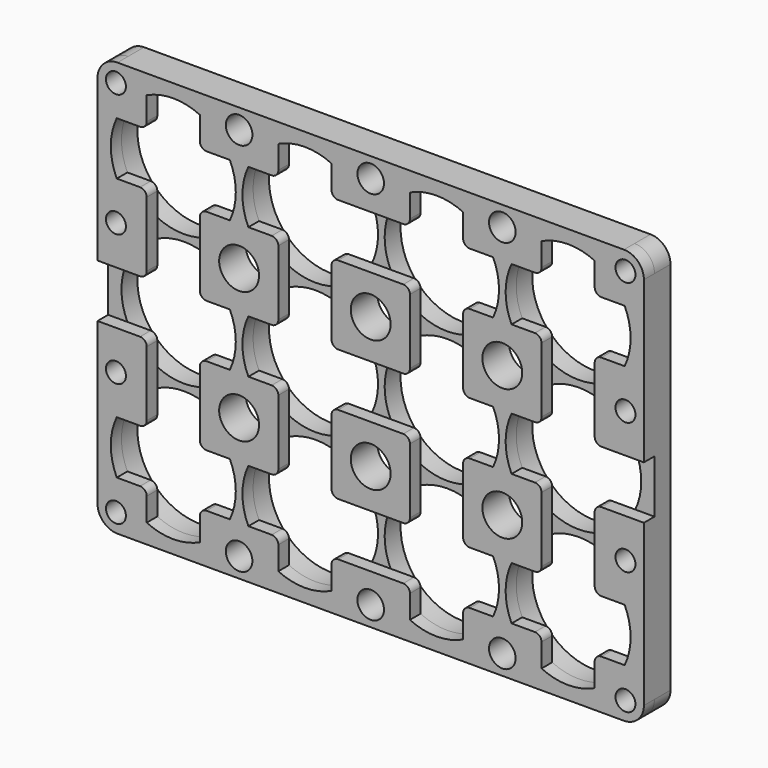
from build123d import *

# Parameters (mm, degrees)
F0_W     = 82.2
F0_H     = 62.4
F0_R     = 1.5
F0_R_2   = 9.4
F0_R_3   = 2
F0_R_4   = 3
F1_DEPTH = 3
F2_R     = 3
F3_R     = 1.5
F3_R_2   = 2
F3_R_3   = 3
F4_DEPTH = 2
F5_R     = 1


# Not quite as in the source:
# - after a boolean that leaves OpenCascade's solid faulty, fix() repairs it


with BuildPart() as f1:
    # F0 (on Front) → F1 (new body)
    with BuildSketch(Plane.XZ):
        with Locations((29.7, 19.8)):
            Rectangle(F0_W, F0_H)
        with Locations((-8.630645927, -8.630645927)):
            Circle(F0_R, mode=Mode.SUBTRACT)
        Circle(F0_R_2, mode=Mode.SUBTRACT)
        with Locations((9.9, -8.4255563615)):
            Circle(F0_R_3, mode=Mode.SUBTRACT)
        with Locations((19.8, 0)):
            Circle(F0_R_2, mode=Mode.SUBTRACT)
        with Locations((-8.630645927, 9.9)):
            Circle(F0_R, mode=Mode.SUBTRACT)
        with Locations((9.9, 9.9)):
            Circle(F0_R_4, mode=Mode.SUBTRACT)
        with Locations((29.7, -8.4255563615)):
            Circle(F0_R_3, mode=Mode.SUBTRACT)
        with Locations((49.5, -8.4255563615)):
            Circle(F0_R_3, mode=Mode.SUBTRACT)
        with Locations((39.6, 0)):
            Circle(F0_R_2, mode=Mode.SUBTRACT)
        with Locations((68.030645927, -8.630645927)):
            Circle(F0_R, mode=Mode.SUBTRACT)
        with Locations((59.4, 0)):
            Circle(F0_R_2, mode=Mode.SUBTRACT)
        with Locations((29.7, 9.9)):
            Circle(F0_R_4, mode=Mode.SUBTRACT)
        with Locations((49.5, 9.9)):
            Circle(F0_R_4, mode=Mode.SUBTRACT)
        with Locations((68.030645927, 9.9)):
            Circle(F0_R, mode=Mode.SUBTRACT)
        with Locations((0, 19.8)):
            Circle(F0_R_2, mode=Mode.SUBTRACT)
        with Locations((-8.630645927, 29.7)):
            Circle(F0_R, mode=Mode.SUBTRACT)
        with Locations((19.8, 19.8)):
            Circle(F0_R_2, mode=Mode.SUBTRACT)
        with Locations((9.9, 29.7)):
            Circle(F0_R_4, mode=Mode.SUBTRACT)
        with Locations((0, 39.6)):
            Circle(F0_R_2, mode=Mode.SUBTRACT)
        with Locations((-8.630645927, 48.230645927)):
            Circle(F0_R, mode=Mode.SUBTRACT)
        with Locations((19.8, 39.6)):
            Circle(F0_R_2, mode=Mode.SUBTRACT)
        with Locations((9.9, 48.0255563615)):
            Circle(F0_R_3, mode=Mode.SUBTRACT)
        with Locations((39.6, 19.8)):
            Circle(F0_R_2, mode=Mode.SUBTRACT)
        with Locations((29.7, 29.7)):
            Circle(F0_R_4, mode=Mode.SUBTRACT)
        with Locations((49.5, 29.7)):
            Circle(F0_R_4, mode=Mode.SUBTRACT)
        with Locations((59.4, 19.8)):
            Circle(F0_R_2, mode=Mode.SUBTRACT)
        with Locations((68.030645927, 29.7)):
            Circle(F0_R, mode=Mode.SUBTRACT)
        with Locations((39.6, 39.6)):
            Circle(F0_R_2, mode=Mode.SUBTRACT)
        with Locations((29.7, 48.0255563615)):
            Circle(F0_R_3, mode=Mode.SUBTRACT)
        with Locations((49.5, 48.0255563615)):
            Circle(F0_R_3, mode=Mode.SUBTRACT)
        with Locations((59.4, 39.6)):
            Circle(F0_R_2, mode=Mode.SUBTRACT)
        with Locations((68.030645927, 48.230645927)):
            Circle(F0_R, mode=Mode.SUBTRACT)
    extrude(amount=F1_DEPTH)

    # F2
    f2_edges = [f1.edges().sort_by_distance(p)[0] for p in [
        (70.8, -1.5, 51),
        (-11.4, -1.5, 51),
        (-11.4, -1.5, -11.4),
        (70.8, -1.5, -11.4),
    ]]
    fillet(f2_edges, radius=F2_R)

    # F3 (on face) → F4 (join)
    with BuildSketch(Plane.XZ.offset(3)):
        with BuildLine():
            ThreePointArc((70.8, 48), (69.9213203436, 50.1213203436), (67.8, 51))
            Line((67.8, 51), (63.4, 51))
            Line((63.4, 51), (63.4, 48.1064681273))
            ThreePointArc((63.4, 48.1064681273), (66.0468037432, 46.2468037432), (67.9064681273, 43.6))
            Line((67.9064681273, 43.6), (70.8, 43.6))
            Line((70.8, 43.6), (70.8, 48))
        make_face()
        with Locations((68.030645927, 48.230645927)):
            Circle(F3_R, mode=Mode.SUBTRACT)
        with BuildLine():
            Line((63.4, 48.1064681273), (63.4, 51))
            Line((63.4, 51), (55.4, 51))
            Line((55.4, 51), (55.4, 48.1064681273))
            ThreePointArc((55.4, 48.1064681273), (59.4, 49), (63.4, 48.1064681273))
        make_face()
        with BuildLine():
            Line((55.4, 48.1064681273), (55.4, 51))
            Line((55.4, 51), (43.6, 51))
            Line((43.6, 51), (43.6, 48.1064681273))
            ThreePointArc((43.6, 48.1064681273), (46.2468037432, 46.2468037432), (48.1064681273, 43.6))
            Line((48.1064681273, 43.6), (50.8935318727, 43.6))
            ThreePointArc((50.8935318727, 43.6), (52.7531962568, 46.2468037432), (55.4, 48.1064681273))
        make_face()
        with Locations((49.5, 48.0255563615)):
            Circle(F3_R_2, mode=Mode.SUBTRACT)
        with BuildLine():
            ThreePointArc((67.9064681273, 43.6), (66.0468037432, 46.2468037432), (63.4, 48.1064681273))
            Line((63.4, 48.1064681273), (63.4, 43.6))
            Line((63.4, 43.6), (67.9064681273, 43.6))
        make_face()
        with BuildLine():
            Line((70.8, 39.6), (70.8, 43.6))
            Line((70.8, 43.6), (67.9064681273, 43.6))
            ThreePointArc((67.9064681273, 43.6), (68.5738977648, 41.6492925125), (68.8, 39.6))
            ThreePointArc((68.8, 39.6), (68.5738977648, 37.5507074875), (67.9064681273, 35.6))
            Line((67.9064681273, 35.6), (70.8, 35.6))
            Line((70.8, 35.6), (70.8, 39.6))
        make_face()
        with BuildLine():
            Line((43.6, 48.1064681273), (43.6, 51))
            Line((43.6, 51), (35.6, 51))
            Line((35.6, 51), (35.6, 48.1064681273))
            ThreePointArc((35.6, 48.1064681273), (39.6, 49), (43.6, 48.1064681273))
        make_face()
        with BuildLine():
            Line((55.4, 43.6), (55.4, 48.1064681273))
            ThreePointArc((55.4, 48.1064681273), (52.7531962568, 46.2468037432), (50.8935318727, 43.6))
            Line((50.8935318727, 43.6), (55.4, 43.6))
        make_face()
        with BuildLine():
            Line((35.6, 48.1064681273), (35.6, 51))
            Line((35.6, 51), (23.8, 51))
            Line((23.8, 51), (23.8, 48.1064681273))
            ThreePointArc((23.8, 48.1064681273), (26.4468037432, 46.2468037432), (28.3064681273, 43.6))
            Line((28.3064681273, 43.6), (31.0935318727, 43.6))
            ThreePointArc((31.0935318727, 43.6), (32.9531962568, 46.2468037432), (35.6, 48.1064681273))
        make_face()
        with Locations((29.7, 48.0255563615)):
            Circle(F3_R_2, mode=Mode.SUBTRACT)
        with BuildLine():
            ThreePointArc((48.1064681273, 43.6), (46.2468037432, 46.2468037432), (43.6, 48.1064681273))
            Line((43.6, 48.1064681273), (43.6, 43.6))
            Line((43.6, 43.6), (48.1064681273, 43.6))
        make_face()
        with BuildLine():
            ThreePointArc((50.8935318727, 35.6), (50, 39.6), (50.8935318727, 43.6))
            Line((50.8935318727, 43.6), (48.1064681273, 43.6))
            ThreePointArc((48.1064681273, 43.6), (48.7738977648, 41.6492925125), (49, 39.6))
            ThreePointArc((49, 39.6), (48.7738977648, 37.5507074875), (48.1064681273, 35.6))
            Line((48.1064681273, 35.6), (50.8935318727, 35.6))
        make_face()
        with BuildLine():
            Line((70.8, 23.8), (70.8, 35.6))
            Line((70.8, 35.6), (67.9064681273, 35.6))
            ThreePointArc((67.9064681273, 35.6), (66.0468037432, 32.9531962568), (63.4, 31.0935318727))
            Line((63.4, 31.0935318727), (63.4, 28.3064681273))
            ThreePointArc((63.4, 28.3064681273), (66.0468037432, 26.4468037432), (67.9064681273, 23.8))
            Line((67.9064681273, 23.8), (70.8, 23.8))
        make_face()
        with Locations((68.030645927, 29.7)):
            Circle(F3_R, mode=Mode.SUBTRACT)
        with BuildLine():
            Line((23.8, 48.1064681273), (23.8, 51))
            Line((23.8, 51), (15.8, 51))
            Line((15.8, 51), (15.8, 48.1064681273))
            ThreePointArc((15.8, 48.1064681273), (19.8, 49), (23.8, 48.1064681273))
        make_face()
        with BuildLine():
            Line((35.6, 43.6), (35.6, 48.1064681273))
            ThreePointArc((35.6, 48.1064681273), (32.9531962568, 46.2468037432), (31.0935318727, 43.6))
            Line((31.0935318727, 43.6), (35.6, 43.6))
        make_face()
        with BuildLine():
            Line((55.4, 35.6), (50.8935318727, 35.6))
            ThreePointArc((50.8935318727, 35.6), (52.7531962568, 32.9531962568), (55.4, 31.0935318727))
            Line((55.4, 31.0935318727), (55.4, 35.6))
        make_face()
        with BuildLine():
            ThreePointArc((55.4, 31.0935318727), (52.7531962568, 32.9531962568), (50.8935318727, 35.6))
            Line((50.8935318727, 35.6), (48.1064681273, 35.6))
            ThreePointArc((48.1064681273, 35.6), (46.2468037432, 32.9531962568), (43.6, 31.0935318727))
            Line((43.6, 31.0935318727), (43.6, 28.3064681273))
            ThreePointArc((43.6, 28.3064681273), (46.2468037432, 26.4468037432), (48.1064681273, 23.8))
            Line((48.1064681273, 23.8), (50.8935318727, 23.8))
            ThreePointArc((50.8935318727, 23.8), (52.7531962568, 26.4468037432), (55.4, 28.3064681273))
            Line((55.4, 28.3064681273), (55.4, 31.0935318727))
        make_face()
        with Locations((49.5, 29.7)):
            Circle(F3_R_3, mode=Mode.SUBTRACT)
        with BuildLine():
            ThreePointArc((63.4, 31.0935318727), (66.0468037432, 32.9531962568), (67.9064681273, 35.6))
            Line((67.9064681273, 35.6), (63.4, 35.6))
            Line((63.4, 35.6), (63.4, 31.0935318727))
        make_face()
        with BuildLine():
            Line((15.8, 48.1064681273), (15.8, 51))
            Line((15.8, 51), (4, 51))
            Line((4, 51), (4, 48.1064681273))
            ThreePointArc((4, 48.1064681273), (6.6468037432, 46.2468037432), (8.5064681273, 43.6))
            Line((8.5064681273, 43.6), (11.2935318727, 43.6))
            ThreePointArc((11.2935318727, 43.6), (13.1531962568, 46.2468037432), (15.8, 48.1064681273))
        make_face()
        with Locations((9.9, 48.0255563615)):
            Circle(F3_R_2, mode=Mode.SUBTRACT)
        with BuildLine():
            ThreePointArc((28.3064681273, 43.6), (26.4468037432, 46.2468037432), (23.8, 48.1064681273))
            Line((23.8, 48.1064681273), (23.8, 43.6))
            Line((23.8, 43.6), (28.3064681273, 43.6))
        make_face()
        with BuildLine():
            ThreePointArc((43.6, 31.0935318727), (46.2468037432, 32.9531962568), (48.1064681273, 35.6))
            Line((48.1064681273, 35.6), (43.6, 35.6))
            Line((43.6, 35.6), (43.6, 31.0935318727))
        make_face()
        with BuildLine():
            Line((70.8, 4), (70.8, 15.8))
            Line((70.8, 15.8), (67.9064681273, 15.8))
            ThreePointArc((67.9064681273, 15.8), (66.0468037432, 13.1531962568), (63.4, 11.2935318727))
            Line((63.4, 11.2935318727), (63.4, 8.5064681273))
            ThreePointArc((63.4, 8.5064681273), (66.0468037432, 6.6468037432), (67.9064681273, 4))
            Line((67.9064681273, 4), (70.8, 4))
        make_face()
        with Locations((68.030645927, 9.9)):
            Circle(F3_R, mode=Mode.SUBTRACT)
        with BuildLine():
            Line((63.4, 23.8), (67.9064681273, 23.8))
            ThreePointArc((67.9064681273, 23.8), (66.0468037432, 26.4468037432), (63.4, 28.3064681273))
            Line((63.4, 28.3064681273), (63.4, 23.8))
        make_face()
        with BuildLine():
            Line((4, 48.1064681273), (4, 51))
            Line((4, 51), (-4, 51))
            Line((-4, 51), (-4, 48.1064681273))
            ThreePointArc((-4, 48.1064681273), (0, 49), (4, 48.1064681273))
        make_face()
        with BuildLine():
            Line((15.8, 43.6), (15.8, 48.1064681273))
            ThreePointArc((15.8, 48.1064681273), (13.1531962568, 46.2468037432), (11.2935318727, 43.6))
            Line((11.2935318727, 43.6), (15.8, 43.6))
        make_face()
        with BuildLine():
            Line((35.6, 35.6), (31.0935318727, 35.6))
            ThreePointArc((31.0935318727, 35.6), (32.9531962568, 32.9531962568), (35.6, 31.0935318727))
            Line((35.6, 31.0935318727), (35.6, 35.6))
        make_face()
        with BuildLine():
            ThreePointArc((35.6, 31.0935318727), (32.9531962568, 32.9531962568), (31.0935318727, 35.6))
            Line((31.0935318727, 35.6), (28.3064681273, 35.6))
            ThreePointArc((28.3064681273, 35.6), (26.4468037432, 32.9531962568), (23.8, 31.0935318727))
            Line((23.8, 31.0935318727), (23.8, 28.3064681273))
            ThreePointArc((23.8, 28.3064681273), (26.4468037432, 26.4468037432), (28.3064681273, 23.8))
            Line((28.3064681273, 23.8), (31.0935318727, 23.8))
            ThreePointArc((31.0935318727, 23.8), (32.9531962568, 26.4468037432), (35.6, 28.3064681273))
            Line((35.6, 28.3064681273), (35.6, 31.0935318727))
        make_face()
        with Locations((29.7, 29.7)):
            Circle(F3_R_3, mode=Mode.SUBTRACT)
        with BuildLine():
            Line((55.4, 23.8), (55.4, 28.3064681273))
            ThreePointArc((55.4, 28.3064681273), (52.7531962568, 26.4468037432), (50.8935318727, 23.8))
            Line((50.8935318727, 23.8), (55.4, 23.8))
        make_face()
        with BuildLine():
            Line((70.8, -4), (70.8, 4))
            Line((70.8, 4), (67.9064681273, 4))
            ThreePointArc((67.9064681273, 4), (68.5738977648, 2.0492925125), (68.8, 0))
            ThreePointArc((68.8, 0), (68.5738977648, -2.0492925125), (67.9064681273, -4))
            Line((67.9064681273, -4), (70.8, -4))
        make_face()
        with BuildLine():
            ThreePointArc((63.4, 11.2935318727), (66.0468037432, 13.1531962568), (67.9064681273, 15.8))
            Line((67.9064681273, 15.8), (63.4, 15.8))
            Line((63.4, 15.8), (63.4, 11.2935318727))
        make_face()
        with BuildLine():
            Line((-4, 48.1064681273), (-4, 51))
            Line((-4, 51), (-8.4, 51))
            ThreePointArc((-8.4, 51), (-10.5213203436, 50.1213203436), (-11.4, 48))
            Line((-11.4, 48), (-11.4, 43.6))
            Line((-11.4, 43.6), (-8.5064681273, 43.6))
            ThreePointArc((-8.5064681273, 43.6), (-6.6468037432, 46.2468037432), (-4, 48.1064681273))
        make_face()
        with Locations((-8.630645927, 48.230645927)):
            Circle(F3_R, mode=Mode.SUBTRACT)
        with BuildLine():
            ThreePointArc((8.5064681273, 43.6), (6.6468037432, 46.2468037432), (4, 48.1064681273))
            Line((4, 48.1064681273), (4, 43.6))
            Line((4, 43.6), (8.5064681273, 43.6))
        make_face()
        with BuildLine():
            ThreePointArc((11.2935318727, 35.6), (10.4, 39.6), (11.2935318727, 43.6))
            Line((11.2935318727, 43.6), (8.5064681273, 43.6))
            ThreePointArc((8.5064681273, 43.6), (9.1738977648, 41.6492925125), (9.4, 39.6))
            ThreePointArc((9.4, 39.6), (9.1738977648, 37.5507074875), (8.5064681273, 35.6))
            Line((8.5064681273, 35.6), (11.2935318727, 35.6))
        make_face()
        with BuildLine():
            ThreePointArc((23.8, 31.0935318727), (26.4468037432, 32.9531962568), (28.3064681273, 35.6))
            Line((28.3064681273, 35.6), (23.8, 35.6))
            Line((23.8, 35.6), (23.8, 31.0935318727))
        make_face()
        with BuildLine():
            ThreePointArc((50.8935318727, 15.8), (50, 19.8), (50.8935318727, 23.8))
            Line((50.8935318727, 23.8), (48.1064681273, 23.8))
            ThreePointArc((48.1064681273, 23.8), (48.7738977648, 21.8492925125), (49, 19.8))
            ThreePointArc((49, 19.8), (48.7738977648, 17.7507074875), (48.1064681273, 15.8))
            Line((48.1064681273, 15.8), (50.8935318727, 15.8))
        make_face()
        with BuildLine():
            ThreePointArc((48.1064681273, 23.8), (46.2468037432, 26.4468037432), (43.6, 28.3064681273))
            Line((43.6, 28.3064681273), (43.6, 23.8))
            Line((43.6, 23.8), (48.1064681273, 23.8))
        make_face()
        with BuildLine():
            Line((70.8, -8.4), (70.8, -4))
            Line((70.8, -4), (67.9064681273, -4))
            ThreePointArc((67.9064681273, -4), (66.0468037432, -6.6468037432), (63.4, -8.5064681273))
            Line((63.4, -8.5064681273), (63.4, -11.4))
            Line((63.4, -11.4), (67.8, -11.4))
            ThreePointArc((67.8, -11.4), (69.9213203436, -10.5213203436), (70.8, -8.4))
        make_face()
        with Locations((68.030645927, -8.630645927)):
            Circle(F3_R, mode=Mode.SUBTRACT)
        with BuildLine():
            Line((63.4, 4), (67.9064681273, 4))
            ThreePointArc((67.9064681273, 4), (66.0468037432, 6.6468037432), (63.4, 8.5064681273))
            Line((63.4, 8.5064681273), (63.4, 4))
        make_face()
        with BuildLine():
            Line((-4, 43.6), (-4, 48.1064681273))
            ThreePointArc((-4, 48.1064681273), (-6.6468037432, 46.2468037432), (-8.5064681273, 43.6))
            Line((-8.5064681273, 43.6), (-4, 43.6))
        make_face()
        with BuildLine():
            Line((15.8, 35.6), (11.2935318727, 35.6))
            ThreePointArc((11.2935318727, 35.6), (13.1531962568, 32.9531962568), (15.8, 31.0935318727))
            Line((15.8, 31.0935318727), (15.8, 35.6))
        make_face()
        with BuildLine():
            ThreePointArc((15.8, 31.0935318727), (13.1531962568, 32.9531962568), (11.2935318727, 35.6))
            Line((11.2935318727, 35.6), (8.5064681273, 35.6))
            ThreePointArc((8.5064681273, 35.6), (6.6468037432, 32.9531962568), (4, 31.0935318727))
            Line((4, 31.0935318727), (4, 28.3064681273))
            ThreePointArc((4, 28.3064681273), (6.6468037432, 26.4468037432), (8.5064681273, 23.8))
            Line((8.5064681273, 23.8), (11.2935318727, 23.8))
            ThreePointArc((11.2935318727, 23.8), (13.1531962568, 26.4468037432), (15.8, 28.3064681273))
            Line((15.8, 28.3064681273), (15.8, 31.0935318727))
        make_face()
        with Locations((9.9, 29.7)):
            Circle(F3_R_3, mode=Mode.SUBTRACT)
        with BuildLine():
            Line((35.6, 23.8), (35.6, 28.3064681273))
            ThreePointArc((35.6, 28.3064681273), (32.9531962568, 26.4468037432), (31.0935318727, 23.8))
            Line((31.0935318727, 23.8), (35.6, 23.8))
        make_face()
        with BuildLine():
            Line((55.4, 15.8), (50.8935318727, 15.8))
            ThreePointArc((50.8935318727, 15.8), (52.7531962568, 13.1531962568), (55.4, 11.2935318727))
            Line((55.4, 11.2935318727), (55.4, 15.8))
        make_face()
        with BuildLine():
            ThreePointArc((55.4, 11.2935318727), (52.7531962568, 13.1531962568), (50.8935318727, 15.8))
            Line((50.8935318727, 15.8), (48.1064681273, 15.8))
            ThreePointArc((48.1064681273, 15.8), (46.2468037432, 13.1531962568), (43.6, 11.2935318727))
            Line((43.6, 11.2935318727), (43.6, 8.5064681273))
            ThreePointArc((43.6, 8.5064681273), (46.2468037432, 6.6468037432), (48.1064681273, 4))
            Line((48.1064681273, 4), (50.8935318727, 4))
            ThreePointArc((50.8935318727, 4), (52.7531962568, 6.6468037432), (55.4, 8.5064681273))
            Line((55.4, 8.5064681273), (55.4, 11.2935318727))
        make_face()
        with Locations((49.5, 9.9)):
            Circle(F3_R_3, mode=Mode.SUBTRACT)
        with BuildLine():
            ThreePointArc((63.4, -8.5064681273), (66.0468037432, -6.6468037432), (67.9064681273, -4))
            Line((67.9064681273, -4), (63.4, -4))
            Line((63.4, -4), (63.4, -8.5064681273))
        make_face()
        with BuildLine():
            ThreePointArc((-8.5064681273, 35.6), (-9.4, 39.6), (-8.5064681273, 43.6))
            Line((-8.5064681273, 43.6), (-11.4, 43.6))
            Line((-11.4, 43.6), (-11.4, 39.6))
            Line((-11.4, 39.6), (-11.4, 35.6))
            Line((-11.4, 35.6), (-8.5064681273, 35.6))
        make_face()
        with BuildLine():
            ThreePointArc((4, 31.0935318727), (6.6468037432, 32.9531962568), (8.5064681273, 35.6))
            Line((8.5064681273, 35.6), (4, 35.6))
            Line((4, 35.6), (4, 31.0935318727))
        make_face()
        with BuildLine():
            ThreePointArc((28.3064681273, 23.8), (26.4468037432, 26.4468037432), (23.8, 28.3064681273))
            Line((23.8, 28.3064681273), (23.8, 23.8))
            Line((23.8, 23.8), (28.3064681273, 23.8))
        make_face()
        with BuildLine():
            ThreePointArc((43.6, 11.2935318727), (46.2468037432, 13.1531962568), (48.1064681273, 15.8))
            Line((48.1064681273, 15.8), (43.6, 15.8))
            Line((43.6, 15.8), (43.6, 11.2935318727))
        make_face()
        with BuildLine():
            Line((63.4, -11.4), (63.4, -8.5064681273))
            ThreePointArc((63.4, -8.5064681273), (59.4, -9.4), (55.4, -8.5064681273))
            Line((55.4, -8.5064681273), (55.4, -11.4))
            Line((55.4, -11.4), (63.4, -11.4))
        make_face()
        with BuildLine():
            Line((55.4, 4), (55.4, 8.5064681273))
            ThreePointArc((55.4, 8.5064681273), (52.7531962568, 6.6468037432), (50.8935318727, 4))
            Line((50.8935318727, 4), (55.4, 4))
        make_face()
        with BuildLine():
            ThreePointArc((-4, 31.0935318727), (-6.6468037432, 32.9531962568), (-8.5064681273, 35.6))
            Line((-8.5064681273, 35.6), (-11.4, 35.6))
            Line((-11.4, 35.6), (-11.4, 23.8))
            Line((-11.4, 23.8), (-8.5064681273, 23.8))
            ThreePointArc((-8.5064681273, 23.8), (-6.6468037432, 26.4468037432), (-4, 28.3064681273))
            Line((-4, 28.3064681273), (-4, 31.0935318727))
        make_face()
        with Locations((-8.630645927, 29.7)):
            Circle(F3_R, mode=Mode.SUBTRACT)
        with BuildLine():
            Line((-4, 35.6), (-8.5064681273, 35.6))
            ThreePointArc((-8.5064681273, 35.6), (-6.6468037432, 32.9531962568), (-4, 31.0935318727))
            Line((-4, 31.0935318727), (-4, 35.6))
        make_face()
        with BuildLine():
            Line((15.8, 23.8), (15.8, 28.3064681273))
            ThreePointArc((15.8, 28.3064681273), (13.1531962568, 26.4468037432), (11.2935318727, 23.8))
            Line((11.2935318727, 23.8), (15.8, 23.8))
        make_face()
        with BuildLine():
            Line((35.6, 15.8), (31.0935318727, 15.8))
            ThreePointArc((31.0935318727, 15.8), (32.9531962568, 13.1531962568), (35.6, 11.2935318727))
            Line((35.6, 11.2935318727), (35.6, 15.8))
        make_face()
        with BuildLine():
            ThreePointArc((35.6, 11.2935318727), (32.9531962568, 13.1531962568), (31.0935318727, 15.8))
            Line((31.0935318727, 15.8), (28.3064681273, 15.8))
            ThreePointArc((28.3064681273, 15.8), (26.4468037432, 13.1531962568), (23.8, 11.2935318727))
            Line((23.8, 11.2935318727), (23.8, 8.5064681273))
            ThreePointArc((23.8, 8.5064681273), (26.4468037432, 6.6468037432), (28.3064681273, 4))
            Line((28.3064681273, 4), (31.0935318727, 4))
            ThreePointArc((31.0935318727, 4), (32.9531962568, 6.6468037432), (35.6, 8.5064681273))
            Line((35.6, 8.5064681273), (35.6, 11.2935318727))
        make_face()
        with Locations((29.7, 9.9)):
            Circle(F3_R_3, mode=Mode.SUBTRACT)
        with BuildLine():
            Line((55.4, -11.4), (55.4, -8.5064681273))
            ThreePointArc((55.4, -8.5064681273), (52.7531962568, -6.6468037432), (50.8935318727, -4))
            Line((50.8935318727, -4), (48.1064681273, -4))
            ThreePointArc((48.1064681273, -4), (46.2468037432, -6.6468037432), (43.6, -8.5064681273))
            Line((43.6, -8.5064681273), (43.6, -11.4))
            Line((43.6, -11.4), (55.4, -11.4))
        make_face()
        with Locations((49.5, -8.4255563615)):
            Circle(F3_R_2, mode=Mode.SUBTRACT)
        with BuildLine():
            ThreePointArc((50.8935318727, -4), (52.7531962568, -6.6468037432), (55.4, -8.5064681273))
            Line((55.4, -8.5064681273), (55.4, -4))
            Line((55.4, -4), (50.8935318727, -4))
        make_face()
        with BuildLine():
            ThreePointArc((50.8935318727, -4), (50, 0), (50.8935318727, 4))
            Line((50.8935318727, 4), (48.1064681273, 4))
            ThreePointArc((48.1064681273, 4), (48.7738977648, 2.0492925125), (49, 0))
            ThreePointArc((49, 0), (48.7738977648, -2.0492925125), (48.1064681273, -4))
            Line((48.1064681273, -4), (50.8935318727, -4))
        make_face()
        with BuildLine():
            ThreePointArc((11.2935318727, 15.8), (10.4, 19.8), (11.2935318727, 23.8))
            Line((11.2935318727, 23.8), (8.5064681273, 23.8))
            ThreePointArc((8.5064681273, 23.8), (9.1738977648, 21.8492925125), (9.4, 19.8))
            ThreePointArc((9.4, 19.8), (9.1738977648, 17.7507074875), (8.5064681273, 15.8))
            Line((8.5064681273, 15.8), (11.2935318727, 15.8))
        make_face()
        with BuildLine():
            ThreePointArc((8.5064681273, 23.8), (6.6468037432, 26.4468037432), (4, 28.3064681273))
            Line((4, 28.3064681273), (4, 23.8))
            Line((4, 23.8), (8.5064681273, 23.8))
        make_face()
        with BuildLine():
            ThreePointArc((23.8, 11.2935318727), (26.4468037432, 13.1531962568), (28.3064681273, 15.8))
            Line((28.3064681273, 15.8), (23.8, 15.8))
            Line((23.8, 15.8), (23.8, 11.2935318727))
        make_face()
        with BuildLine():
            ThreePointArc((48.1064681273, 4), (46.2468037432, 6.6468037432), (43.6, 8.5064681273))
            Line((43.6, 8.5064681273), (43.6, 4))
            Line((43.6, 4), (48.1064681273, 4))
        make_face()
        with BuildLine():
            Line((-4, 23.8), (-4, 28.3064681273))
            ThreePointArc((-4, 28.3064681273), (-6.6468037432, 26.4468037432), (-8.5064681273, 23.8))
            Line((-8.5064681273, 23.8), (-4, 23.8))
        make_face()
        with BuildLine():
            Line((15.8, 15.8), (11.2935318727, 15.8))
            ThreePointArc((11.2935318727, 15.8), (13.1531962568, 13.1531962568), (15.8, 11.2935318727))
            Line((15.8, 11.2935318727), (15.8, 15.8))
        make_face()
        with BuildLine():
            ThreePointArc((15.8, 11.2935318727), (13.1531962568, 13.1531962568), (11.2935318727, 15.8))
            Line((11.2935318727, 15.8), (8.5064681273, 15.8))
            ThreePointArc((8.5064681273, 15.8), (6.6468037432, 13.1531962568), (4, 11.2935318727))
            Line((4, 11.2935318727), (4, 8.5064681273))
            ThreePointArc((4, 8.5064681273), (6.6468037432, 6.6468037432), (8.5064681273, 4))
            Line((8.5064681273, 4), (11.2935318727, 4))
            ThreePointArc((11.2935318727, 4), (13.1531962568, 6.6468037432), (15.8, 8.5064681273))
            Line((15.8, 8.5064681273), (15.8, 11.2935318727))
        make_face()
        with Locations((9.9, 9.9)):
            Circle(F3_R_3, mode=Mode.SUBTRACT)
        with BuildLine():
            Line((35.6, 4), (35.6, 8.5064681273))
            ThreePointArc((35.6, 8.5064681273), (32.9531962568, 6.6468037432), (31.0935318727, 4))
            Line((31.0935318727, 4), (35.6, 4))
        make_face()
        with BuildLine():
            Line((35.6, -11.4), (43.6, -11.4))
            Line((43.6, -11.4), (43.6, -8.5064681273))
            ThreePointArc((43.6, -8.5064681273), (39.6, -9.4), (35.6, -8.5064681273))
            Line((35.6, -8.5064681273), (35.6, -11.4))
        make_face()
        with BuildLine():
            ThreePointArc((43.6, -8.5064681273), (46.2468037432, -6.6468037432), (48.1064681273, -4))
            Line((48.1064681273, -4), (43.6, -4))
            Line((43.6, -4), (43.6, -8.5064681273))
        make_face()
        with BuildLine():
            Line((-8.5064681273, 15.8), (-11.4, 15.8))
            Line((-11.4, 15.8), (-11.4, 4))
            Line((-11.4, 4), (-8.5064681273, 4))
            ThreePointArc((-8.5064681273, 4), (-6.6468037432, 6.6468037432), (-4, 8.5064681273))
            Line((-4, 8.5064681273), (-4, 11.2935318727))
            ThreePointArc((-4, 11.2935318727), (-6.6468037432, 13.1531962568), (-8.5064681273, 15.8))
        make_face()
        with Locations((-8.630645927, 9.9)):
            Circle(F3_R, mode=Mode.SUBTRACT)
        with BuildLine():
            ThreePointArc((4, 11.2935318727), (6.6468037432, 13.1531962568), (8.5064681273, 15.8))
            Line((8.5064681273, 15.8), (4, 15.8))
            Line((4, 15.8), (4, 11.2935318727))
        make_face()
        with BuildLine():
            ThreePointArc((28.3064681273, 4), (26.4468037432, 6.6468037432), (23.8, 8.5064681273))
            Line((23.8, 8.5064681273), (23.8, 4))
            Line((23.8, 4), (28.3064681273, 4))
        make_face()
        with BuildLine():
            Line((23.8, -11.4), (35.6, -11.4))
            Line((35.6, -11.4), (35.6, -8.5064681273))
            ThreePointArc((35.6, -8.5064681273), (32.9531962568, -6.6468037432), (31.0935318727, -4))
            Line((31.0935318727, -4), (28.3064681273, -4))
            ThreePointArc((28.3064681273, -4), (26.4468037432, -6.6468037432), (23.8, -8.5064681273))
            Line((23.8, -8.5064681273), (23.8, -11.4))
        make_face()
        with Locations((29.7, -8.4255563615)):
            Circle(F3_R_2, mode=Mode.SUBTRACT)
        with BuildLine():
            Line((-8.5064681273, 4), (-11.4, 4))
            Line((-11.4, 4), (-11.4, -4))
            Line((-11.4, -4), (-8.5064681273, -4))
            ThreePointArc((-8.5064681273, -4), (-9.4, 0), (-8.5064681273, 4))
        make_face()
        with BuildLine():
            Line((-4, 15.8), (-8.5064681273, 15.8))
            ThreePointArc((-8.5064681273, 15.8), (-6.6468037432, 13.1531962568), (-4, 11.2935318727))
            Line((-4, 11.2935318727), (-4, 15.8))
        make_face()
        with BuildLine():
            Line((15.8, 4), (15.8, 8.5064681273))
            ThreePointArc((15.8, 8.5064681273), (13.1531962568, 6.6468037432), (11.2935318727, 4))
            Line((11.2935318727, 4), (15.8, 4))
        make_face()
        with BuildLine():
            Line((35.6, -4), (31.0935318727, -4))
            ThreePointArc((31.0935318727, -4), (32.9531962568, -6.6468037432), (35.6, -8.5064681273))
            Line((35.6, -8.5064681273), (35.6, -4))
        make_face()
        with BuildLine():
            Line((15.8, -11.4), (23.8, -11.4))
            Line((23.8, -11.4), (23.8, -8.5064681273))
            ThreePointArc((23.8, -8.5064681273), (19.8, -9.4), (15.8, -8.5064681273))
            Line((15.8, -8.5064681273), (15.8, -11.4))
        make_face()
        with BuildLine():
            Line((-8.5064681273, -4), (-11.4, -4))
            Line((-11.4, -4), (-11.4, -8.4))
            ThreePointArc((-11.4, -8.4), (-10.5213203436, -10.5213203436), (-8.4, -11.4))
            Line((-8.4, -11.4), (-4, -11.4))
            Line((-4, -11.4), (-4, -8.5064681273))
            ThreePointArc((-4, -8.5064681273), (-6.6468037432, -6.6468037432), (-8.5064681273, -4))
        make_face()
        with Locations((-8.630645927, -8.630645927)):
            Circle(F3_R, mode=Mode.SUBTRACT)
        with BuildLine():
            ThreePointArc((-4, 8.5064681273), (-6.6468037432, 6.6468037432), (-8.5064681273, 4))
            Line((-8.5064681273, 4), (-4, 4))
            Line((-4, 4), (-4, 8.5064681273))
        make_face()
        with BuildLine():
            ThreePointArc((11.2935318727, -4), (10.4, 0), (11.2935318727, 4))
            Line((11.2935318727, 4), (8.5064681273, 4))
            ThreePointArc((8.5064681273, 4), (9.1738977648, 2.0492925125), (9.4, 0))
            ThreePointArc((9.4, 0), (9.1738977648, -2.0492925125), (8.5064681273, -4))
            Line((8.5064681273, -4), (11.2935318727, -4))
        make_face()
        with BuildLine():
            ThreePointArc((8.5064681273, 4), (6.6468037432, 6.6468037432), (4, 8.5064681273))
            Line((4, 8.5064681273), (4, 4))
            Line((4, 4), (8.5064681273, 4))
        make_face()
        with BuildLine():
            ThreePointArc((23.8, -8.5064681273), (26.4468037432, -6.6468037432), (28.3064681273, -4))
            Line((28.3064681273, -4), (23.8, -4))
            Line((23.8, -4), (23.8, -8.5064681273))
        make_face()
        with BuildLine():
            Line((4, -11.4), (15.8, -11.4))
            Line((15.8, -11.4), (15.8, -8.5064681273))
            ThreePointArc((15.8, -8.5064681273), (13.1531962568, -6.6468037432), (11.2935318727, -4))
            Line((11.2935318727, -4), (8.5064681273, -4))
            ThreePointArc((8.5064681273, -4), (6.6468037432, -6.6468037432), (4, -8.5064681273))
            Line((4, -8.5064681273), (4, -11.4))
        make_face()
        with Locations((9.9, -8.4255563615)):
            Circle(F3_R_2, mode=Mode.SUBTRACT)
        with BuildLine():
            Line((-4, -4), (-8.5064681273, -4))
            ThreePointArc((-8.5064681273, -4), (-6.6468037432, -6.6468037432), (-4, -8.5064681273))
            Line((-4, -8.5064681273), (-4, -4))
        make_face()
        with BuildLine():
            Line((15.8, -4), (11.2935318727, -4))
            ThreePointArc((11.2935318727, -4), (13.1531962568, -6.6468037432), (15.8, -8.5064681273))
            Line((15.8, -8.5064681273), (15.8, -4))
        make_face()
        with BuildLine():
            Line((-4, -11.4), (4, -11.4))
            Line((4, -11.4), (4, -8.5064681273))
            ThreePointArc((4, -8.5064681273), (0, -9.4), (-4, -8.5064681273))
            Line((-4, -8.5064681273), (-4, -11.4))
        make_face()
        with BuildLine():
            ThreePointArc((4, -8.5064681273), (6.6468037432, -6.6468037432), (8.5064681273, -4))
            Line((8.5064681273, -4), (4, -4))
            Line((4, -4), (4, -8.5064681273))
        make_face()
    extrude(amount=F4_DEPTH)

    add(f1.part.fix(), mode=Mode.REPLACE)

    # F5
    f5_edges = [f1.edges().sort_by_distance(p)[0] for p in [
        (-4, -4, 43.6),
        (4, -4, 43.6),
        (15.8, -4, 43.6),
        (23.8, -4, 43.6),
        (35.6, -4, 43.6),
        (43.6, -4, 43.6),
        (55.4, -4, 43.6),
        (63.4, -4, 43.6),
        (63.4, -4, 23.8),
        (55.4, -4, 23.8),
        (43.6, -4, 23.8),
        (35.6, -4, 23.8),
        (15.8, -4, 23.8),
        (23.8, -4, 23.8),
        (-4, -4, 23.8),
        (4, -4, 23.8),
        (-4, -4, 15.8),
        (-4, -4, 4),
        (4, -4, 4),
        (15.8, -4, 4),
        (15.8, -4, 15.8),
        (23.8, -4, 4),
        (35.6, -4, 4),
        (35.6, -4, 15.8),
        (43.6, -4, 4),
        (55.4, -4, 4),
        (63.4, -4, 4),
        (55.4, -4, 15.8),
        (55.4, -4, -4),
        (-4, -4, -4),
        (4, -4, -4),
        (15.8, -4, -4),
        (23.8, -4, -4),
        (35.6, -4, -4),
        (43.6, -4, -4),
        (63.4, -4, -4),
        (63.4, -4, 15.8),
        (43.6, -4, 15.8),
        (23.8, -4, 15.8),
        (4, -4, 15.8),
        (43.6, -4, 35.6),
        (55.4, -4, 35.6),
        (63.4, -4, 35.6),
        (35.6, -4, 35.6),
        (-4, -4, 35.6),
        (4, -4, 35.6),
        (15.8, -4, 35.6),
        (23.8, -4, 35.6),
    ]]
    fillet(f5_edges, radius=F5_R)


solid = f1.part
